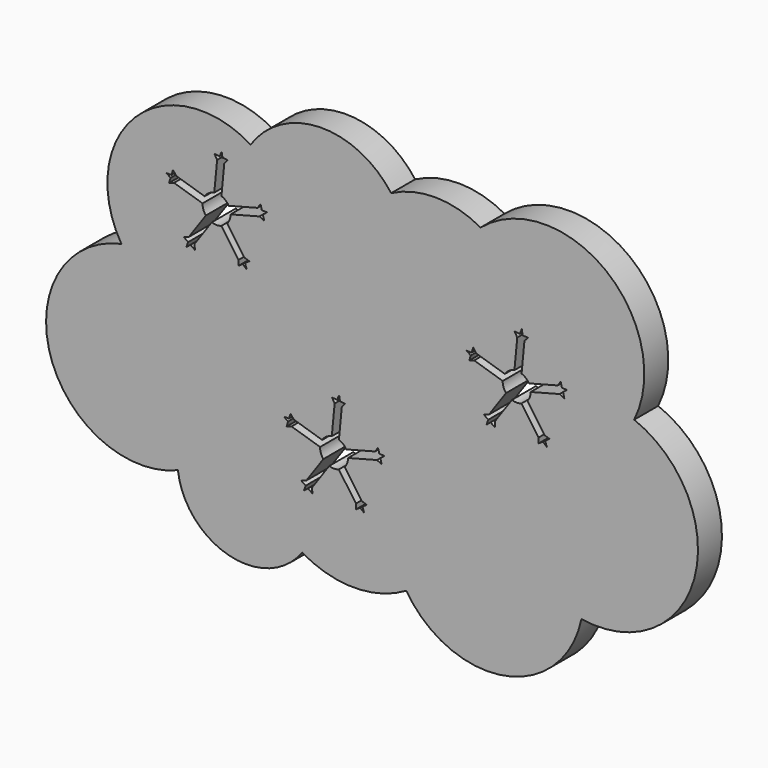
from build123d import *

# Parameters (mm, degrees)
F1_DEPTH = 6.35


# Not quite as in the source:
# - a length typed as a fraction of an inch, garbled in the dataset ("3 / 203.2 mm" for 3/8 in), is restored


with BuildPart() as f1:
    # F0 (on Front) → F1 (new body)
    with BuildSketch(Plane.XZ):
        with BuildLine():
            ThreePointArc((24.579061552, 28.3529026657), (9.5195561517, 35.7531570559), (-5.2125295141, 27.720839839))
            ThreePointArc((-5.2125295141, 27.720839839), (-29.7447728029, 24.816757347), (-32.6261176355, 0.281833099))
            ThreePointArc((-32.6261176355, 0.281833099), (-47.6586884842, -25.465181848), (-20.6299769397, -38.0483339671))
            ThreePointArc((-20.6299769397, -38.0483339671), (-9.7842016961, -50.4339494071), (5.705863164, -44.8579112888))
            ThreePointArc((5.705863164, -44.8579112888), (16.7493256027, -47.8238039479), (27.779373908, -44.8084074092))
            ThreePointArc((27.779373908, -44.8084074092), (48.6340616912, -53.8941801606), (64.9161967707, -38.0082950333))
            ThreePointArc((64.9161967707, -38.0082950333), (88.8664062791, -22.618688114), (76.0994801139, 2.8265105082))
            ThreePointArc((76.0994801139, 2.8265105082), (70.0975710942, 28.7139027136), (43.5306278663, 28.0994805429))
            ThreePointArc((43.5306278663, 28.0994805429), (34.0869435906, 30.6266295541), (24.579061552, 28.3529026657))
        make_face()
        with BuildLine():
            ThreePointArc((9.9552140403, -22.4611988481), (10.8253405255, -21.564938524), (11.9872140403, -21.1061873886))
            Line((11.9872140403, -21.1061873886), (12.5920123004, -14.8077944269))
            Line((12.5920123004, -14.8077944269), (12.0265549094, -13.8484140251))
            Line((12.0265549094, -13.8484140251), (13.1350774738, -13.9548590377))
            Line((13.1350774738, -13.9548590377), (13.5390697269, -12.9171003587))
            Line((13.5390697269, -12.9171003587), (13.7382008585, -14.0127734892))
            Line((13.7382008585, -14.0127734892), (14.8467234229, -14.1192185018))
            Line((14.8467234229, -14.1192185018), (14.1090343836, -14.9534652864))
            Line((14.1090343836, -14.9534652864), (13.5042361235, -21.2518582481))
            ThreePointArc((13.5042361235, -21.2518582481), (14.3943138922, -21.7735734557), (15.0519583946, -22.5685130135))
            Line((15.0519583946, -22.5685130135), (21.1719606568, -20.9619305704))
            Line((21.1719606568, -20.9619305704), (21.788173451, -20.0343344251))
            Line((21.788173451, -20.0343344251), (22.0579849941, -21.114776255))
            Line((22.0579849941, -21.114776255), (23.1710785379, -21.1490629746))
            Line((23.1710785379, -21.1490629746), (22.2940630935, -21.8353549873))
            Line((22.2940630935, -21.8353549873), (22.5638746366, -22.9157968171))
            Line((22.5638746366, -22.9157968171), (21.5589198477, -22.4359857202))
            Line((21.5589198477, -22.4359857202), (15.4389175856, -24.0425681633))
            ThreePointArc((15.4389175856, -24.0425681633), (15.2565271687, -25.0580281222), (14.7374718125, -25.9496596209))
            Line((14.7374718125, -25.9496596209), (18.3579193376, -31.1388690552))
            Line((18.3579193376, -31.1388690552), (19.4102498473, -31.5032188374))
            Line((19.4102498473, -31.5032188374), (18.4969454746, -32.1404200522))
            Line((18.4969454746, -32.1404200522), (18.8616543221, -33.1926261736))
            Line((18.8616543221, -33.1926261736), (18.0000377843, -32.487099982))
            Line((18.0000377843, -32.487099982), (17.0867334116, -33.1243011968))
            Line((17.0867334116, -33.1243011968), (17.1080536411, -32.0108849615))
            Line((17.1080536411, -32.0108849615), (13.487606116, -26.8216755271))
            ThreePointArc((13.487606116, -26.8216755271), (12.471606116, -27.0010332485), (11.455606116, -26.8216755271))
            Line((11.455606116, -26.8216755271), (7.835158591, -32.0108849615))
            Line((7.835158591, -32.0108849615), (7.8564698266, -33.124301369))
            Line((7.8564698266, -33.124301369), (6.9431654539, -32.4871001542))
            Line((6.9431654539, -32.4871001542), (6.0815366025, -33.1926113076))
            Line((6.0815366025, -33.1926113076), (6.4462638144, -32.1404115518))
            Line((6.4462638144, -32.1404115518), (5.5329594417, -31.5032103369))
            Line((5.5329594417, -31.5032103369), (6.5852928945, -31.1388690552))
            Line((6.5852928945, -31.1388690552), (10.2057404195, -25.9496596209))
            ThreePointArc((10.2057404195, -25.9496596209), (9.6657394654, -24.9991764128), (9.5065515642, -23.9176596209))
            Line((9.5065515642, -23.9176596209), (3.4595978764, -22.0548966372))
            Line((3.4595978764, -22.0548966372), (2.4058730089, -22.4152268431))
            Line((2.4058730089, -22.4152268431), (2.7337236859, -21.3509487369))
            Line((2.7337236859, -21.3509487369), (1.7987755438, -20.7459314434))
            Line((1.7987755438, -20.7459314434), (2.9121035894, -20.7719048279))
            Line((2.9121035894, -20.7719048279), (3.2399542664, -19.7076267216))
            Line((3.2399542664, -19.7076267216), (3.9082603526, -20.5984358645))
            Line((3.9082603526, -20.5984358645), (9.9552140403, -22.4611988481))
        make_face(mode=Mode.SUBTRACT)
        with BuildLine():
            ThreePointArc((-14.9548382666, 14.9038782153), (-14.0847117815, 15.8001385395), (-12.9228382666, 16.2588896749))
            Line((-12.9228382666, 16.2588896749), (-12.3180400065, 22.5572826366))
            Line((-12.3180400065, 22.5572826366), (-12.8834973975, 23.5166630384))
            Line((-12.8834973975, 23.5166630384), (-11.7749748332, 23.4102180258))
            Line((-11.7749748332, 23.4102180258), (-11.37098258, 24.4479767047))
            Line((-11.37098258, 24.4479767047), (-11.1718514484, 23.3523035743))
            Line((-11.1718514484, 23.3523035743), (-10.0633288841, 23.2458585617))
            Line((-10.0633288841, 23.2458585617), (-10.8010179234, 22.411611777))
            Line((-10.8010179234, 22.411611777), (-11.4058161835, 16.1132188153))
            ThreePointArc((-11.4058161835, 16.1132188153), (-10.5157384147, 15.5915036078), (-9.8580939123, 14.7965640499))
            Line((-9.8580939123, 14.7965640499), (-3.7380916502, 16.4031464931))
            Line((-3.7380916502, 16.4031464931), (-3.121878856, 17.3307426383))
            Line((-3.121878856, 17.3307426383), (-2.8520673129, 16.2503008085))
            Line((-2.8520673129, 16.2503008085), (-1.7389737691, 16.2160140888))
            Line((-1.7389737691, 16.2160140888), (-2.6159892135, 15.5297220761))
            Line((-2.6159892135, 15.5297220761), (-2.3461776704, 14.4492802463))
            Line((-2.3461776704, 14.4492802463), (-3.3511324592, 14.9290913433))
            Line((-3.3511324592, 14.9290913433), (-9.4711347214, 13.3225089001))
            ThreePointArc((-9.4711347214, 13.3225089001), (-9.6535251382, 12.3070489413), (-10.1725804944, 11.4154174426))
            Line((-10.1725804944, 11.4154174426), (-6.5521329694, 6.2262080082))
            Line((-6.5521329694, 6.2262080082), (-5.4998024597, 5.8618582261))
            Line((-5.4998024597, 5.8618582261), (-6.4131068324, 5.2246570112))
            Line((-6.4131068324, 5.2246570112), (-6.0483979848, 4.1724508898))
            Line((-6.0483979848, 4.1724508898), (-6.9100145227, 4.8779770815))
            Line((-6.9100145227, 4.8779770815), (-7.8233188953, 4.2407758666))
            Line((-7.8233188953, 4.2407758666), (-7.8019986659, 5.354192102))
            Line((-7.8019986659, 5.354192102), (-11.4224461909, 10.5434015363))
            ThreePointArc((-11.4224461909, 10.5434015363), (-12.4384461909, 10.3640438149), (-13.4544461909, 10.5434015363))
            Line((-13.4544461909, 10.5434015363), (-17.0748937159, 5.354192102))
            Line((-17.0748937159, 5.354192102), (-17.0535824803, 4.2407756944))
            Line((-17.0535824803, 4.2407756944), (-17.966886853, 4.8779769093))
            Line((-17.966886853, 4.8779769093), (-18.8285157045, 4.1724657558))
            Line((-18.8285157045, 4.1724657558), (-18.4637884925, 5.2246655117))
            Line((-18.4637884925, 5.2246655117), (-19.3770928652, 5.8618667265))
            Line((-19.3770928652, 5.8618667265), (-18.3247594124, 6.2262080082))
            Line((-18.3247594124, 6.2262080082), (-14.7043118874, 11.4154174426))
            ThreePointArc((-14.7043118874, 11.4154174426), (-15.2443128415, 12.3659006506), (-15.4035007427, 13.4474174426))
            Line((-15.4035007427, 13.4474174426), (-21.4504544305, 15.3101804262))
            Line((-21.4504544305, 15.3101804262), (-22.5041792981, 14.9498502204))
            Line((-22.5041792981, 14.9498502204), (-22.176328621, 16.0141283266))
            Line((-22.176328621, 16.0141283266), (-23.1112767632, 16.61914562))
            Line((-23.1112767632, 16.61914562), (-21.9979487176, 16.5931722356))
            Line((-21.9979487176, 16.5931722356), (-21.6700980405, 17.6574503418))
            Line((-21.6700980405, 17.6574503418), (-21.0017919544, 16.7666411989))
            Line((-21.0017919544, 16.7666411989), (-14.9548382666, 14.9038782153))
        make_face(mode=Mode.SUBTRACT)
        with BuildLine():
            ThreePointArc((48.6740988512, 2.4488521783), (49.5442253363, 3.3451125024), (50.7060988512, 3.8038636378))
            Line((50.7060988512, 3.8038636378), (51.3108971112, 10.1022565995))
            Line((51.3108971112, 10.1022565995), (50.7454397202, 11.0616370013))
            Line((50.7454397202, 11.0616370013), (51.8539622846, 10.9551919887))
            Line((51.8539622846, 10.9551919887), (52.2579545378, 11.9929506677))
            Line((52.2579545378, 11.9929506677), (52.4570856693, 10.8972775372))
            Line((52.4570856693, 10.8972775372), (53.5656082337, 10.7908325246))
            Line((53.5656082337, 10.7908325246), (52.8279191944, 9.95658574))
            Line((52.8279191944, 9.95658574), (52.2231209343, 3.6581927783))
            ThreePointArc((52.2231209343, 3.6581927783), (53.113198703, 3.1364775707), (53.7708432054, 2.3415380128))
            Line((53.7708432054, 2.3415380128), (59.8908454676, 3.948120456))
            Line((59.8908454676, 3.948120456), (60.5070582618, 4.8757166012))
            Line((60.5070582618, 4.8757166012), (60.7768698049, 3.7952747714))
            Line((60.7768698049, 3.7952747714), (61.8899633487, 3.7609880518))
            Line((61.8899633487, 3.7609880518), (61.0129479043, 3.0746960391))
            Line((61.0129479043, 3.0746960391), (61.2827594474, 1.9942542093))
            Line((61.2827594474, 1.9942542093), (60.2778046585, 2.4740653062))
            Line((60.2778046585, 2.4740653062), (54.1578023964, 0.8674828631))
            ThreePointArc((54.1578023964, 0.8674828631), (53.9754119795, -0.1479770958), (53.4563566233, -1.0396085945))
            Line((53.4563566233, -1.0396085945), (57.0768041484, -6.2288180289))
            Line((57.0768041484, -6.2288180289), (58.1291346581, -6.593167811))
            Line((58.1291346581, -6.593167811), (57.2158302854, -7.2303690258))
            Line((57.2158302854, -7.2303690258), (57.5805391329, -8.2825751472))
            Line((57.5805391329, -8.2825751472), (56.7189225951, -7.5770489556))
            Line((56.7189225951, -7.5770489556), (55.8056182224, -8.2142501704))
            Line((55.8056182224, -8.2142501704), (55.8269384519, -7.1008339351))
            Line((55.8269384519, -7.1008339351), (52.2064909269, -1.9116245007))
            ThreePointArc((52.2064909269, -1.9116245007), (51.1904909269, -2.0909822221), (50.1744909269, -1.9116245007))
            Line((50.1744909269, -1.9116245007), (46.5540434018, -7.1008339351))
            Line((46.5540434018, -7.1008339351), (46.5753546374, -8.2142503426))
            Line((46.5753546374, -8.2142503426), (45.6620502647, -7.5770491278))
            Line((45.6620502647, -7.5770491278), (44.8004214133, -8.2825602812))
            Line((44.8004214133, -8.2825602812), (45.1651486252, -7.2303605254))
            Line((45.1651486252, -7.2303605254), (44.2518442526, -6.5931593106))
            Line((44.2518442526, -6.5931593106), (45.3041777053, -6.2288180289))
            Line((45.3041777053, -6.2288180289), (48.9246252304, -1.0396085945))
            ThreePointArc((48.9246252304, -1.0396085945), (48.3846242762, -0.0891253865), (48.225436375, 0.9923914055))
            Line((48.225436375, 0.9923914055), (42.1784826873, 2.8551543891))
            Line((42.1784826873, 2.8551543891), (41.1247578197, 2.4948241833))
            Line((41.1247578197, 2.4948241833), (41.4526084967, 3.5591022895))
            Line((41.4526084967, 3.5591022895), (40.5176603546, 4.164119583))
            Line((40.5176603546, 4.164119583), (41.6309884002, 4.1381461985))
            Line((41.6309884002, 4.1381461985), (41.9588390772, 5.2024243047))
            Line((41.9588390772, 5.2024243047), (42.6271451634, 4.3116151619))
            Line((42.6271451634, 4.3116151619), (48.6740988512, 2.4488521783))
        make_face(mode=Mode.SUBTRACT)
    extrude(amount=F1_DEPTH)


solid = f1.part
